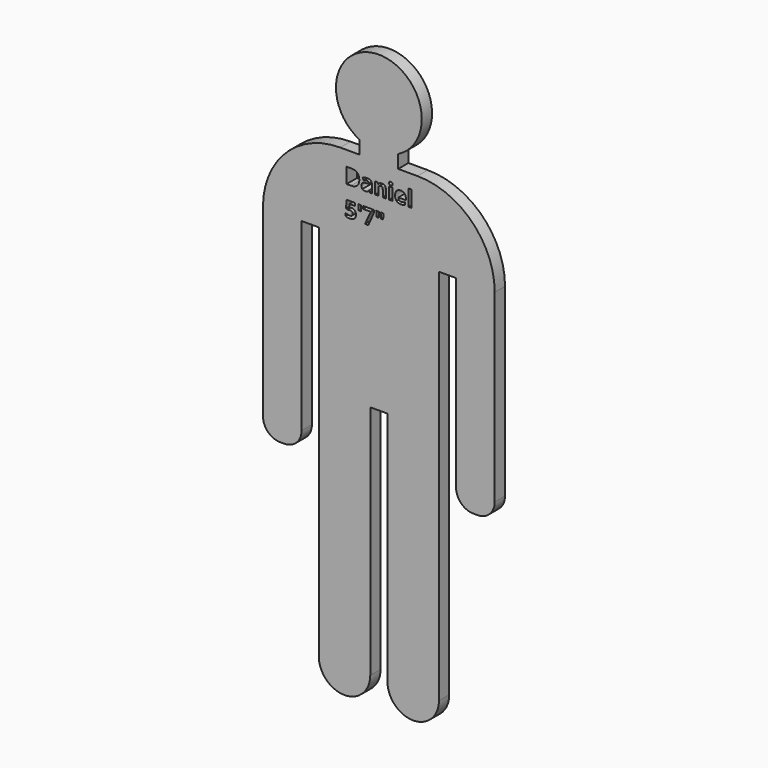
from build123d import *

# Parameters (mm, degrees)
F0_W     = 9.4439018923
F0_H     = 34.6243370532
F0_H_2   = 48.1906557211
F1_DEPTH = 38.1


with BuildPart() as f1:
    # F0 (on Front) → F1 (new body)
    with BuildSketch(Plane.XZ):
        with BuildLine():
            Line((48.0189776897, 759.9984430313), (48.0189776897, 798.9838165495))
            ThreePointArc((48.0189776897, 798.9838165495), (-9.1310223103, 1039.3984430313), (-66.2810223103, 798.9838165495))
            Line((-66.2810223103, 798.9838165495), (-66.2810223103, 759.9984430313))
            Line((-66.2810223103, 759.9984430313), (-123.4310223103, 759.9984430313))
            ThreePointArc((-123.4310223103, 759.9984430313), (-285.0756324895, 693.0430532106), (-352.0310223103, 531.3984430313))
            Line((-352.0310223103, 531.3984430313), (-352.0310223103, -14.7015569687))
            ThreePointArc((-352.0310223103, -14.7015569687), (-337.1520467945, -50.622581453), (-301.2310223103, -65.5015569687))
            Line((-301.2310223103, -65.5015569687), (-288.5310223103, -65.5015569687))
            ThreePointArc((-288.5310223103, -65.5015569687), (-252.609997826, -50.622581453), (-237.7310223103, -14.7015569687))
            Line((-237.7310223103, -14.7015569687), (-237.7310223103, 531.3984430313))
            Line((-237.7310223103, 531.3984430313), (-186.9310223103, 531.3984430313))
            Line((-186.9310223103, 531.3984430313), (-186.9310223103, -586.2015569687))
            ThreePointArc((-186.9310223103, -586.2015569687), (-164.6125590367, -640.0830936951), (-110.7310223103, -662.4015569687))
            ThreePointArc((-110.7310223103, -662.4015569687), (-56.8494855838, -640.0830936951), (-34.5310223103, -586.2015569687))
            Line((-34.5310223103, -586.2015569687), (-34.5310223103, 112.2984430313))
            Line((-34.5310223103, 112.2984430313), (16.2689776897, 112.2984430313))
            Line((16.2689776897, 112.2984430313), (16.2689776897, -586.2015569687))
            ThreePointArc((16.2689776897, -586.2015569687), (38.5874409633, -640.0830936951), (92.4689776897, -662.4015569687))
            ThreePointArc((92.4689776897, -662.4015569687), (146.3505144162, -640.0830936951), (168.6689776897, -586.2015569687))
            Line((168.6689776897, -586.2015569687), (168.6689776897, 531.3984430313))
            Line((168.6689776897, 531.3984430313), (219.4689776897, 531.3984430313))
            Line((219.4689776897, 531.3984430313), (219.4689776897, -14.7015569687))
            ThreePointArc((219.4689776897, -14.7015569687), (234.3479532055, -50.622581453), (270.2689776897, -65.5015569687))
            Line((270.2689776897, -65.5015569687), (282.9689776897, -65.5015569687))
            ThreePointArc((282.9689776897, -65.5015569687), (318.890002174, -50.622581453), (333.7689776897, -14.7015569687))
            Line((333.7689776897, -14.7015569687), (333.7689776897, 531.3984430313))
            ThreePointArc((333.7689776897, 531.3984430313), (266.813587869, 693.0430532106), (105.1689776897, 759.9984430313))
            Line((105.1689776897, 759.9984430313), (48.0189776897, 759.9984430313))
        make_face()
        with BuildLine():
            add(Edge.make_bspline(
                [(-95.9296966802, 613.2359054213), (-94.0369524395, 613.6719302726), (-91.2523391848, 613.6719302726)],
                knots=[0, 0, 0, 1, 1, 1], degree=2))
            add(Edge.make_bspline(
                [(-91.2523391848, 613.6719302726), (-84.6921471043, 613.6719302726), (-80.8026072379, 609.9855383482)],
                knots=[0, 0, 0, 1, 1, 1], degree=2))
            add(Edge.make_bspline(
                [(-80.8026072379, 609.9855383482), (-76.9130673714, 606.2991464238), (-76.9130673714, 599.887599179)],
                knots=[0, 0, 0, 1, 1, 1], degree=2))
            add(Edge.make_bspline(
                [(-76.9130673714, 599.887599179), (-76.9130673714, 592.3067125603), (-81.5904248669, 588.2140247518)],
                knots=[0, 0, 0, 1, 1, 1], degree=2))
            add(Edge.make_bspline(
                [(-81.5904248669, 588.2140247518), (-86.2677823623, 584.1213369433), (-94.9684600763, 584.1213369433)],
                knots=[0, 0, 0, 1, 1, 1], degree=2))
            add(Edge.make_bspline(
                [(-94.9684600763, 584.1213369433), (-102.5295273836, 584.1213369433), (-107.1672462562, 586.5690219038)],
                knots=[0, 0, 0, 1, 1, 1], degree=2))
            Line((-107.1672462562, 586.5690219038), (-107.1672462562, 594.8435844223))
            add(Edge.make_bspline(
                [(-107.1672462562, 594.8435844223), (-104.7294709513, 593.5454195242), (-101.4741490504, 592.7229181002)],
                knots=[0, 0, 0, 1, 1, 1], degree=2))
            add(Edge.make_bspline(
                [(-101.4741490504, 592.7229181002), (-98.2188271494, 591.9004166762), (-95.3152980262, 591.9004166762)],
                knots=[0, 0, 0, 1, 1, 1], degree=2))
            add(Edge.make_bspline(
                [(-95.3152980262, 591.9004166762), (-86.5452527222, 591.9004166762), (-86.5452527222, 599.0849170664)],
                knots=[0, 0, 0, 1, 1, 1], degree=2))
            add(Edge.make_bspline(
                [(-86.5452527222, 599.0849170664), (-86.5452527222, 605.9324891625), (-95.6224973532, 605.9324891625)],
                knots=[0, 0, 0, 1, 1, 1], degree=2))
            add(Edge.make_bspline(
                [(-95.6224973532, 605.9324891625), (-97.2575905455, 605.9324891625), (-99.2395216876, 605.6054705241)],
                knots=[0, 0, 0, 1, 1, 1], degree=2))
            add(Edge.make_bspline(
                [(-99.2395216876, 605.6054705241), (-101.2214528297, 605.2784518856), (-102.4601597936, 604.9018849686)],
                knots=[0, 0, 0, 1, 1, 1], degree=2))
            Line((-102.4601597936, 604.9018849686), (-106.2753772422, 606.9531837007))
            Line((-106.2753772422, 606.9531837007), (-104.57091646, 630.0228621952))
            Line((-104.57091646, 630.0228621952), (-80.0147896089, 630.0228621952))
            Line((-80.0147896089, 630.0228621952), (-80.0147896089, 621.9068541682))
            Line((-80.0147896089, 621.9068541682), (-96.177438073, 621.9068541682))
            Line((-96.177438073, 621.9068541682), (-97.0098491527, 613.0178929957))
            Line((-97.0098491527, 613.0178929957), (-95.9296966802, 613.2359054213))
        make_face(mode=Mode.SUBTRACT)
        Polygon((-40.1284253733, 584.7456452531), (-50.1669066082, 584.7456452531), (-33.1619374087, 621.9068541682), (-55.4883917249, 621.9068541682), (-55.4883917249, 629.963404261), (-23.0045403052, 629.963404261), (-23.0045403052, 623.9482432446), align=None, mode=Mode.SUBTRACT)
        Polygon((-69.9465794068, 630.0228621952), (-61.3053596271, 630.0228621952), (-62.5837052137, 613.6719302726), (-68.6781434758, 613.6719302726), align=None, mode=Mode.SUBTRACT)
        with BuildLine():
            add(Edge.make_bspline(
                [(-73.1374885456, 710.424853804), (-67.0034116607, 704.5732021068), (-67.0034116607, 694.0689670535)],
                knots=[0, 0, 0, 1, 1, 1], degree=2))
            add(Edge.make_bspline(
                [(-67.0034116607, 694.0689670535), (-67.0034116607, 682.8908754118), (-73.3703654548, 676.9450819854)],
                knots=[0, 0, 0, 1, 1, 1], degree=2))
            add(Edge.make_bspline(
                [(-73.3703654548, 676.9450819854), (-79.737319249, 670.999288559), (-91.7478219703, 670.999288559)],
                knots=[0, 0, 0, 1, 1, 1], degree=2))
            Line((-91.7478219703, 670.999288559), (-104.57091646, 670.999288559))
            Line((-104.57091646, 670.999288559), (-104.57091646, 716.2765055011))
            Line((-104.57091646, 716.2765055011), (-90.3604701708, 716.2765055011))
            add(Edge.make_bspline(
                [(-90.3604701708, 716.2765055011), (-79.2715654306, 716.2765055011), (-73.1374885456, 710.424853804)],
                knots=[0, 0, 0, 1, 1, 1], degree=2))
        make_face(mode=Mode.SUBTRACT)
        Polygon((-16.8704634203, 630.0228621952), (-8.2292436406, 630.0228621952), (-9.5075892273, 613.6719302726), (-15.6020274893, 613.6719302726), align=None, mode=Mode.SUBTRACT)
        with BuildLine():
            Line((-29.7827448113, 670.999288559), (-36.372665859, 670.999288559))
            Line((-36.372665859, 670.999288559), (-38.2059521654, 675.7063750215))
            Line((-38.2059521654, 675.7063750215), (-38.4536935582, 675.7063750215))
            add(Edge.make_bspline(
                [(-38.4536935582, 675.7063750215), (-40.8320109288, 672.7037493412), (-43.358973135, 671.5393647952)],
                knots=[0, 0, 0, 1, 1, 1], degree=2))
            add(Edge.make_bspline(
                [(-43.358973135, 671.5393647952), (-45.8859353412, 670.3749802492), (-49.9389845269, 670.3749802492)],
                knots=[0, 0, 0, 1, 1, 1], degree=2))
            add(Edge.make_bspline(
                [(-49.9389845269, 670.3749802492), (-54.9235413494, 670.3749802492), (-57.7874318498, 673.2289610939)],
                knots=[0, 0, 0, 1, 1, 1], degree=2))
            add(Edge.make_bspline(
                [(-57.7874318498, 673.2289610939), (-60.6513223502, 676.0829419385), (-60.6513223502, 681.3449691209)],
                knots=[0, 0, 0, 1, 1, 1], degree=2))
            add(Edge.make_bspline(
                [(-60.6513223502, 681.3449691209), (-60.6513223502, 686.8547376961), (-56.7964662787, 689.4708868037)],
                knots=[0, 0, 0, 1, 1, 1], degree=2))
            add(Edge.make_bspline(
                [(-56.7964662787, 689.4708868037), (-52.9416102072, 692.0870359113), (-45.1724401301, 692.3645062712)],
                knots=[0, 0, 0, 1, 1, 1], degree=2))
            Line((-45.1724401301, 692.3645062712), (-39.1572791137, 692.5527897297))
            Line((-39.1572791137, 692.5527897297), (-39.1572791137, 694.0689670535))
            add(Edge.make_bspline(
                [(-39.1572791137, 694.0689670535), (-39.1572791137, 699.3309942358), (-44.5481318203, 699.3309942358)],
                knots=[0, 0, 0, 1, 1, 1], degree=2))
            add(Edge.make_bspline(
                [(-44.5481318203, 699.3309942358), (-48.7002775631, 699.3309942358), (-54.3091426953, 696.823851341)],
                knots=[0, 0, 0, 1, 1, 1], degree=2))
            Line((-54.3091426953, 696.823851341), (-57.4306842442, 703.2056696187))
            add(Edge.make_bspline(
                [(-57.4306842442, 703.2056696187), (-51.4551618506, 706.3371208233), (-44.181474559, 706.3371208233)],
                knots=[0, 0, 0, 1, 1, 1], degree=2))
            add(Edge.make_bspline(
                [(-44.181474559, 706.3371208233), (-37.2149865944, 706.3371208233), (-33.4988657029, 703.299811348)],
                knots=[0, 0, 0, 1, 1, 1], degree=2))
            add(Edge.make_bspline(
                [(-33.4988657029, 703.299811348), (-29.7827448113, 700.2625018726), (-29.7827448113, 694.0689670535)],
                knots=[0, 0, 0, 1, 1, 1], degree=2))
            Line((-29.7827448113, 694.0689670535), (-29.7827448113, 670.999288559))
        make_face(mode=Mode.SUBTRACT)
        Polygon((-3.8095371936, 630.0228621952), (4.8316825861, 630.0228621952), (3.5632466551, 613.6719302726), (-2.5311916069, 613.6719302726), align=None, mode=Mode.SUBTRACT)
        with BuildLine():
            Line((11.9071767635, 693.5734842679), (11.9071767635, 670.999288559))
            Line((11.9071767635, 670.999288559), (2.4632748713, 670.999288559))
            Line((2.4632748713, 670.999288559), (2.4632748713, 691.2248958645))
            add(Edge.make_bspline(
                [(2.4632748713, 691.2248958645), (2.4632748713, 694.9707457231), (1.1304261782, 696.8436706525)],
                knots=[0, 0, 0, 1, 1, 1], degree=2))
            add(Edge.make_bspline(
                [(1.1304261782, 696.8436706525), (-0.2024225149, 698.7165955818), (-3.1158612939, 698.7165955818)],
                knots=[0, 0, 0, 1, 1, 1], degree=2))
            add(Edge.make_bspline(
                [(-3.1158612939, 698.7165955818), (-7.0797235781, 698.7165955818), (-8.8436422946, 696.070717507)],
                knots=[0, 0, 0, 1, 1, 1], degree=2))
            add(Edge.make_bspline(
                [(-8.8436422946, 696.070717507), (-10.6075610112, 693.4248394323), (-10.6075610112, 687.2907625473)],
                knots=[0, 0, 0, 1, 1, 1], degree=2))
            Line((-10.6075610112, 687.2907625473), (-10.6075610112, 670.999288559))
            Line((-10.6075610112, 670.999288559), (-20.0514629034, 670.999288559))
            Line((-20.0514629034, 670.999288559), (-20.0514629034, 705.6236256121))
            Line((-20.0514629034, 705.6236256121), (-12.8372335461, 705.6236256121))
            Line((-12.8372335461, 705.6236256121), (-11.5687976151, 701.1940095094))
            Line((-11.5687976151, 701.1940095094), (-11.0435858624, 701.1940095094))
            add(Edge.make_bspline(
                [(-11.0435858624, 701.1940095094), (-9.4580409487, 703.7011524043), (-6.6882921776, 704.9844528188)],
                knots=[0, 0, 0, 1, 1, 1], degree=2))
            add(Edge.make_bspline(
                [(-6.6882921776, 704.9844528188), (-3.9185434064, 706.2677532333), (-0.3907059734, 706.2677532333)],
                knots=[0, 0, 0, 1, 1, 1], degree=2))
            add(Edge.make_bspline(
                [(-0.3907059734, 706.2677532333), (5.6541840101, 706.2677532333), (8.7806803868, 703.0025216766)],
                knots=[0, 0, 0, 1, 1, 1], degree=2))
            add(Edge.make_bspline(
                [(8.7806803868, 703.0025216766), (11.9071767635, 699.73729012), (11.9071767635, 693.5734842679)],
                knots=[0, 0, 0, 1, 1, 1], degree=2))
        make_face(mode=Mode.SUBTRACT)
        with Locations((26.3504999619, 688.3114570855)):
            Rectangle(F0_W, F0_H, mode=Mode.SUBTRACT)
        with BuildLine():
            add(Edge.make_bspline(
                [(26.3653644455, 709.9244161906), (21.2222531316, 709.9244161906), (21.2222531316, 714.5720447189)],
                knots=[0, 0, 0, 1, 1, 1], degree=2))
            add(Edge.make_bspline(
                [(21.2222531316, 714.5720447189), (21.2222531316, 719.1899442801), (26.3653644455, 719.1899442801)],
                knots=[0, 0, 0, 1, 1, 1], degree=2))
            add(Edge.make_bspline(
                [(26.3653644455, 719.1899442801), (31.5084757593, 719.1899442801), (31.5084757593, 714.5720447189)],
                knots=[0, 0, 0, 1, 1, 1], degree=2))
            add(Edge.make_bspline(
                [(31.5084757593, 714.5720447189), (31.5084757593, 712.3721011511), (30.2251753448, 711.1482586708)],
                knots=[0, 0, 0, 1, 1, 1], degree=2))
            add(Edge.make_bspline(
                [(30.2251753448, 711.1482586708), (28.9418749302, 709.9244161906), (26.3653644455, 709.9244161906)],
                knots=[0, 0, 0, 1, 1, 1], degree=2))
        make_face(mode=Mode.SUBTRACT)
        with BuildLine():
            add(Edge.make_bspline(
                [(63.5265733606, 670.9794692475), (60.7122311387, 670.3749802492), (56.6492722973, 670.3749802492)],
                knots=[0, 0, 0, 1, 1, 1], degree=2))
            add(Edge.make_bspline(
                [(56.6492722973, 670.3749802492), (48.2954325332, 670.3749802492), (43.5883460706, 674.9928798104)],
                knots=[0, 0, 0, 1, 1, 1], degree=2))
            add(Edge.make_bspline(
                [(43.5883460706, 674.9928798104), (38.8812596081, 679.6107793716), (38.8812596081, 688.0637156928)],
                knots=[0, 0, 0, 1, 1, 1], degree=2))
            add(Edge.make_bspline(
                [(38.8812596081, 688.0637156928), (38.8812596081, 696.7643934068), (43.2315984651, 701.51607332)],
                knots=[0, 0, 0, 1, 1, 1], degree=2))
            add(Edge.make_bspline(
                [(43.2315984651, 701.51607332), (47.5819373221, 706.2677532333), (55.2619204978, 706.2677532333)],
                knots=[0, 0, 0, 1, 1, 1], degree=2))
            add(Edge.make_bspline(
                [(55.2619204978, 706.2677532333), (62.5950657238, 706.2677532333), (66.6827987044, 702.0908333513)],
                knots=[0, 0, 0, 1, 1, 1], degree=2))
            add(Edge.make_bspline(
                [(66.6827987044, 702.0908333513), (70.7705316851, 697.9139134692), (70.7705316851, 690.5411296205)],
                knots=[0, 0, 0, 1, 1, 1], degree=2))
            Line((70.7705316851, 690.5411296205), (70.7705316851, 685.9529590264))
            Line((70.7705316851, 685.9529590264), (48.4440773689, 685.9529590264))
            add(Edge.make_bspline(
                [(48.4440773689, 685.9529590264), (48.6026318603, 681.9296388079), (50.8323043952, 679.6702373058)],
                knots=[0, 0, 0, 1, 1, 1], degree=2))
            add(Edge.make_bspline(
                [(50.8323043952, 679.6702373058), (53.0619769301, 677.4108358038), (57.0852971486, 677.4108358038)],
                knots=[0, 0, 0, 1, 1, 1], degree=2))
            add(Edge.make_bspline(
                [(57.0852971486, 677.4108358038), (60.2167483532, 677.4108358038), (63.0013616079, 678.0599182528)],
                knots=[0, 0, 0, 1, 1, 1], degree=2))
            add(Edge.make_bspline(
                [(63.0013616079, 678.0599182528), (65.7859748626, 678.7090007019), (68.8183295101, 680.1359911242)],
                knots=[0, 0, 0, 1, 1, 1], degree=2))
            Line((68.8183295101, 680.1359911242), (68.8183295101, 672.8226652097))
            add(Edge.make_bspline(
                [(68.8183295101, 672.8226652097), (66.3409155824, 671.5839582459), (63.5265733606, 670.9794692475)],
                knots=[0, 0, 0, 1, 1, 1], degree=2))
        make_face(mode=Mode.SUBTRACT)
        with Locations((83.172465807, 695.0946164195)):
            Rectangle(F0_W, F0_H_2, mode=Mode.SUBTRACT)
    extrude(amount=F1_DEPTH)


solid = f1.part
